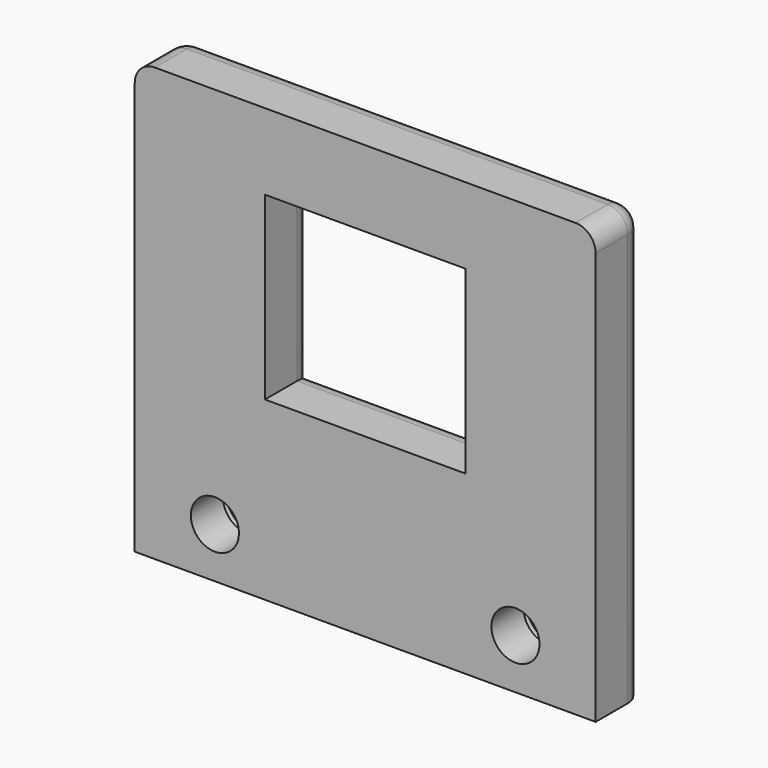
from build123d import *

# Parameters (mm, degrees)
F0_W           = 6.5
F0_H           = 5
F0_W_2         = 10
F0_H_2         = 9
F1_DEPTH       = 3
F2_D           = 2.4
F2_DEPTH       = 3
F2_CBORE_D     = 4
F2_CBORE_DEPTH = 1
F2_TIP         = 0.7210327428
F3_R           = 1


# Not quite as in the source:
# - a feature names something its author has since deleted; it is built from what else it names


with BuildPart() as f1:
    # F0 (on Front) → F1 (new body)
    with BuildSketch(Plane.XZ):
        with Locations((8.25, -8.3)):
            Rectangle(F0_W, F0_H)
        with Locations((0, -8.3)):
            Rectangle(F0_W_2, F0_H)
        with Locations((-8.25, -8.3)):
            Rectangle(F0_W, F0_H)
        Polygon((5, -5.8), (11.5, -5.8), (11.5, 10.8), (-11.5, 10.8), (-11.5, -5.8), (-5, -5.8), align=None)
        with Locations((0, 2.5)):
            Rectangle(F0_W_2, F0_H_2, mode=Mode.SUBTRACT)
    extrude(amount=F1_DEPTH)

    # F2
    with Locations(Plane(origin=(0, 0, 0), x_dir=(1, 0, 0), z_dir=(0, 1, 0))):
        with Locations((7.5, 8.3), (-7.5, 8.3)):
            CounterBoreHole(F2_D / 2, F2_CBORE_D / 2, F2_CBORE_DEPTH, depth=F2_DEPTH)
            with Locations((0, 0, -(F2_DEPTH + F2_TIP / 2))):  # 118° drill point
                Cone(0, F2_D / 2, F2_TIP, mode=Mode.SUBTRACT)

    # F3
    f3_edges = [f1.edges().sort_by_distance(p)[0] for p in [
        (-11.5, 0, 0),
        (0, 0, 10.8),
        (11.5, -1.5, 10.8),
        (-11.5, -1.5, 10.8),
        (11.5, 0, 0),
        (-5, 0, 2.5),
        (0, 0, 7),
        (5, 0, 2.5),
        (0, 0, -2),
    ]]
    fillet(f3_edges, radius=F3_R)


solid = f1.part
